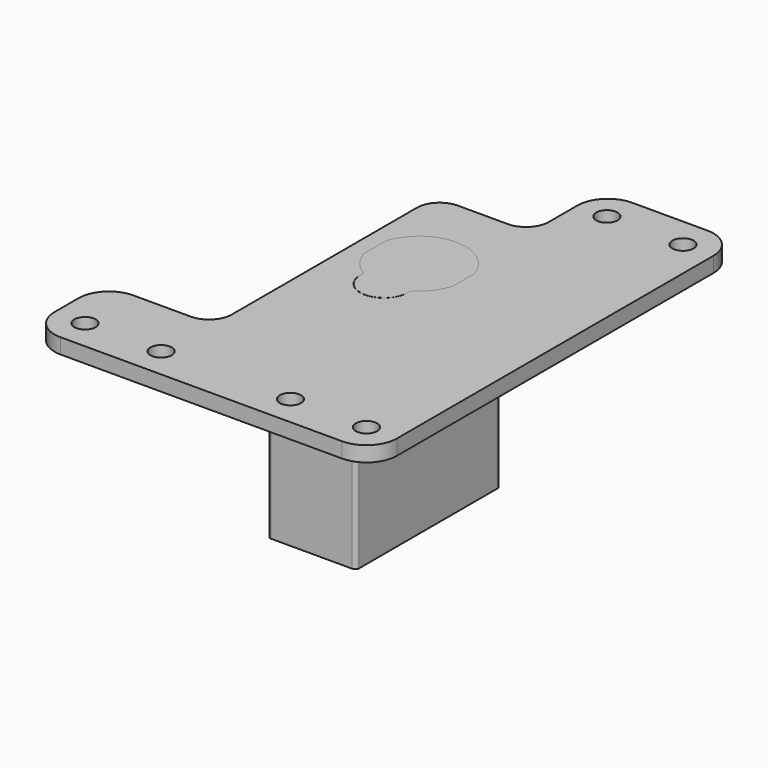
from build123d import *

# Parameters (mm, degrees)
F0_W     = 11.65
F0_H     = 23.75
F1_DEPTH = 20.4
F3_DEPTH = 6
F5_START = -0.8
F4_W     = 11.65
F4_H     = 4.2
F5_DEPTH = 2
F6_R     = 0.5
F7_R     = 1
F8_R     = 1.4
F9_DEPTH = 2
F10_R    = 4


with BuildPart() as f1:
    # F0 (on Top) → F1 (new body)
    with BuildSketch(Plane.XY):
        Rectangle(F0_W, F0_H)
    extrude(amount=F1_DEPTH)

    # F2 (on face) → F3 (join)
    with BuildSketch(Plane.XY.offset(20.4)):
        with BuildLine():
            Line((5.825, 3.9640955299), (5.825, 7.5859044701))
            ThreePointArc((5.825, 7.5859044701), (0, 11.875), (-5.825, 7.5859044701))
            Line((-5.825, 7.5859044701), (-5.825, 3.9640955299))
            ThreePointArc((-5.825, 3.9640955299), (-4.7781429098, 1.9829886164), (-3.0865775367, 0.5135326087))
            ThreePointArc((-3.0865775367, 0.5135326087), (0, -3.1), (3.0865775367, 0.5135326087))
            ThreePointArc((3.0865775367, 0.5135326087), (4.7781429098, 1.9829886164), (5.825, 3.9640955299))
        make_face()
    extrude(amount=F3_DEPTH)

    # F4 (on face) → F5 (join)
    with BuildSketch(Plane.XY.offset(20.4).offset(F5_START)):
        with Locations((0, -13.975)):
            Rectangle(F4_W, F4_H)
        with Locations((0, 13.975)):
            Rectangle(F4_W, F4_H)
    extrude(amount=-F5_DEPTH)

    # F6
    f6_edges = [f1.edges().sort_by_distance(p)[0] for p in [
        (5.825, 11.875, 8.8),
        (5.825, -11.875, 8.8),
        (-5.825, -11.875, 8.8),
        (-5.825, 11.875, 8.8),
    ]]
    fillet(f6_edges, radius=F6_R)

    # F7
    f7_edges = [f1.edges().sort_by_distance(p)[0] for p in [
        (-5.825, 16.075, 18.6),
        (5.825, 16.075, 18.6),
        (5.825, -16.075, 18.6),
        (-5.825, -16.075, 18.6),
    ]]
    fillet(f7_edges, radius=F7_R)


with BuildPart() as f9:
    # F8 (on face) → F9 (new body)
    with BuildSketch(Plane.XY.offset(26.4)):
        with BuildLine():
            Line((22.5, -30), (22.5, 30))
            Line((22.5, 30), (4.6129450202, 30))
            Line((4.6129450202, 30), (4.6129450202, 21.3236394078))
            ThreePointArc((4.6129450202, 21.3236394078), (3.7342653638, 19.2023190642), (1.6129450202, 18.3236394078))
            Line((1.6129450202, 18.3236394078), (-4.9445159063, 18.3236394078))
            ThreePointArc((-4.9445159063, 18.3236394078), (-7.0658362498, 17.4449597513), (-7.9445159063, 15.3236394078))
            Line((-7.9445159063, 15.3236394078), (-7.9445159063, -15.0673655123))
            ThreePointArc((-7.9445159063, -15.0673655123), (-8.8231955627, -17.1886858558), (-10.9445159063, -18.0673655123))
            Line((-10.9445159063, -18.0673655123), (-22.5, -18.0673655123))
            Line((-22.5, -18.0673655123), (-22.5, -30))
            Line((-22.5, -30), (22.5, -30))
        make_face()
        with Locations((-18.5, -26)):
            Circle(F8_R, mode=Mode.SUBTRACT)
        with Locations((-8.5, -26)):
            Circle(F8_R, mode=Mode.SUBTRACT)
        with Locations((8.5, -26)):
            Circle(F8_R, mode=Mode.SUBTRACT)
        with Locations((18.5, -26)):
            Circle(F8_R, mode=Mode.SUBTRACT)
        with BuildLine():
            ThreePointArc((5.825, 3.9640955299), (4.7781429098, 1.9829886164), (3.0865775367, 0.5135326087))
            ThreePointArc((3.0865775367, 0.5135326087), (0, -3.1290056936), (-3.0865775367, 0.5135326087))
            ThreePointArc((-3.0865775367, 0.5135326087), (-4.7781429098, 1.9829886164), (-5.825, 3.9640955299))
            Line((-5.825, 3.9640955299), (-5.825, 7.5859044701))
            ThreePointArc((-5.825, 7.5859044701), (0, 11.875), (5.825, 7.5859044701))
            Line((5.825, 7.5859044701), (5.825, 3.9640955299))
        make_face(mode=Mode.SUBTRACT)
        with Locations((8.5, 26)):
            Circle(F8_R, mode=Mode.SUBTRACT)
        with Locations((18.5, 26)):
            Circle(F8_R, mode=Mode.SUBTRACT)
    extrude(amount=-F9_DEPTH)

    # F10
    f10_edges = [f9.edges().sort_by_distance(p)[0] for p in [
        (-22.5, -30, 25.4),
        (22.5, 30, 25.4),
        (22.5, -30, 25.4),
        (4.612945, 30, 25.4),
        (-22.5, -18.067366, 25.4),
    ]]
    fillet(f10_edges, radius=F10_R)


with BuildPart() as f11_1:
    # F11: copy of F9
    add(f9.part)


solid = Compound([f1.part, f9.part])
